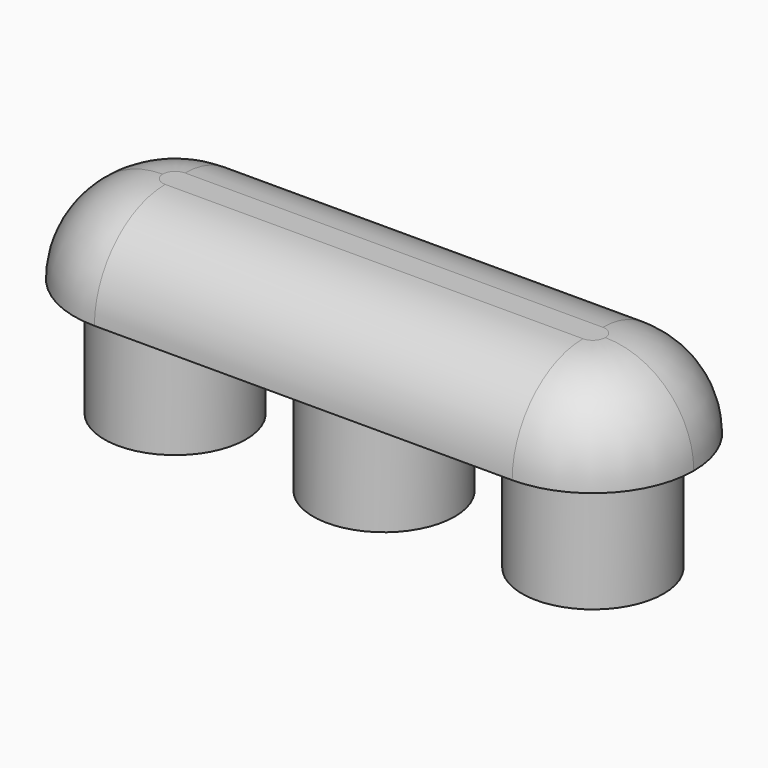
from build123d import *

# Parameters (mm, degrees)
F0_R     = 6
F1_DEPTH = 7.5
F2_DEPTH = 10
F3_R     = 7.49999


# Not quite as in the source:
# - a fillet or chamfer is up to 0.001 mm smaller than in the source, because OpenCascade refuses the exact size


with BuildPart() as f1:
    # F0 (on Top) → F1 (new body)
    with BuildSketch(Plane.XY):
        with BuildLine():
            Line((-17.8126084931, 40.3974354923), (-53.2126084931, 40.3974354923))
            ThreePointArc((-53.2126084931, 40.3974354923), (-59.2583714722, 37.8931984714), (-61.7626084931, 31.8474354923))
            ThreePointArc((-61.7626084931, 31.8474354923), (-59.2583714722, 25.8016725131), (-53.2126084931, 23.2974354923))
            Line((-53.2126084931, 23.2974354923), (-17.8126084931, 23.2974354923))
            ThreePointArc((-17.8126084931, 23.2974354923), (-11.7668455139, 25.8016725131), (-9.2626084931, 31.8474354923))
            ThreePointArc((-9.2626084931, 31.8474354923), (-11.7668455139, 37.8931984714), (-17.8126084931, 40.3974354923))
        make_face()
        with Locations((-53.2126084931, 31.8474354923)):
            Circle(F0_R, mode=Mode.SUBTRACT)
        with Locations((-35.5126084931, 31.8474354923)):
            Circle(F0_R, mode=Mode.SUBTRACT)
        with Locations((-17.8126084931, 31.8474354923)):
            Circle(F0_R, mode=Mode.SUBTRACT)
        with Locations((-53.2126084931, 31.8474354923)):
            Circle(F0_R)
        with Locations((-35.5126084931, 31.8474354923)):
            Circle(F0_R)
        with Locations((-17.8126084931, 31.8474354923)):
            Circle(F0_R)
    extrude(amount=F1_DEPTH)

    # F0 (on Top) → F2 (join)
    with BuildSketch(Plane.XY):
        with Locations((-53.2126084931, 31.8474354923)):
            Circle(F0_R)
        with Locations((-35.5126084931, 31.8474354923)):
            Circle(F0_R)
        with Locations((-17.8126084931, 31.8474354923)):
            Circle(F0_R)
    extrude(amount=-F2_DEPTH)

    # F3 (radius 7.5 in the source; OpenCascade refuses exactly that, so slightly less here)
    f3_edges = [f1.edges().sort_by_distance(p)[0] for p in [
        (-61.762608, 31.847435, 7.5),
    ]]
    fillet(f3_edges, radius=F3_R)


solid = f1.part
